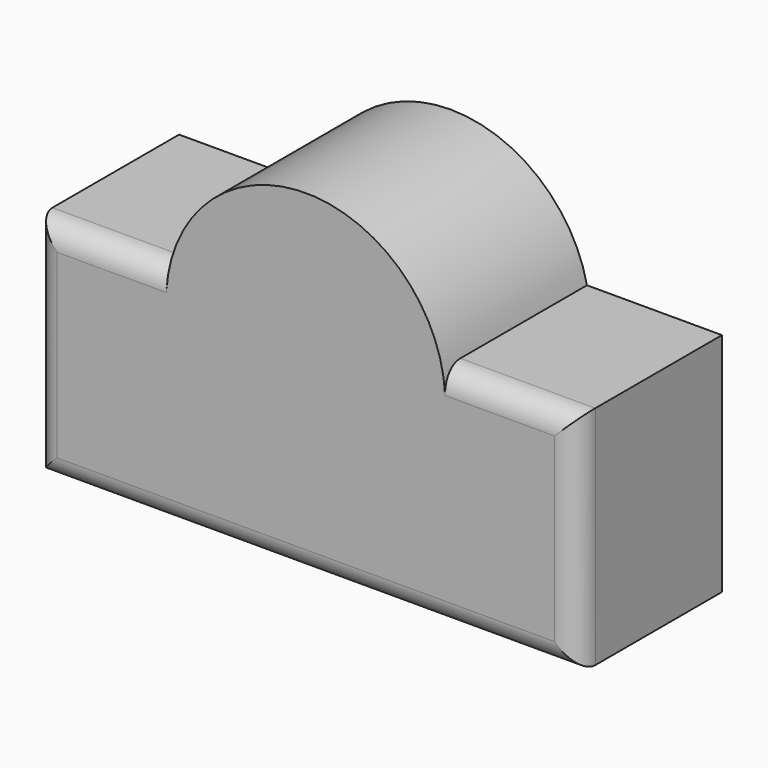
from build123d import *

# Parameters (mm, degrees)
F1_DEPTH = 40
F2_R     = 450
F3_DEPTH = 25
F4_R     = 5


with BuildPart() as f1:
    # F0 (on Front) → F1 (new body)
    with BuildSketch(Plane.XZ):
        Polygon((-60, -25), (60, -25), (60, 25), (30.1694516093, 25), (-30.1694516093, 25), (-60, 25), align=None)
        with BuildLine():
            Line((-30.1694516093, 25), (30.1694516093, 25))
            ThreePointArc((30.1694516093, 25), (0, 49.4079397137), (-30.1694516093, 25))
        make_face()
    extrude(amount=F1_DEPTH)

    # F2 (on face) → F3 (cut)
    with BuildSketch(Plane.XZ.offset(40)):
        Circle(F2_R)
        with BuildLine():
            Line((60, -25), (-60, -25))
            Line((-60, -25), (-60, 25))
            Line((-60, 25), (-30.1694516093, 25))
            ThreePointArc((-30.1694516093, 25), (0, 49.4079397137), (30.1694516093, 25))
            Line((30.1694516093, 25), (60, 25))
            Line((60, 25), (60, -25))
        make_face(mode=Mode.SUBTRACT)
    extrude(amount=-F3_DEPTH, mode=Mode.SUBTRACT)

    # F4
    f4_edges = [f1.edges().sort_by_distance(p)[0] for p in [
        (-60, -40, 0),
        (45.084726, -40, 25),
        (-45.084726, -40, 25),
        (60, -40, 0),
        (0, -40, -25),
    ]]
    fillet(f4_edges, radius=F4_R)


solid = f1.part
